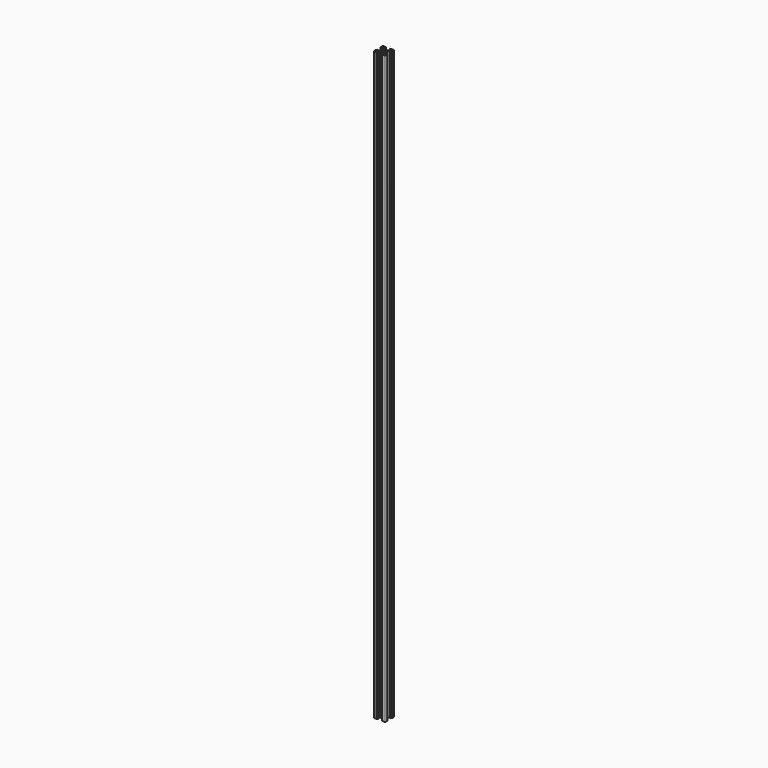
from build123d import *

# Parameters (mm, degrees)
F0_R     = 2.09999979
F1_DEPTH = 1000


# Not quite as in the source:
# - ends of sketch curves that miss each other by under 0.0002 mm in the source are joined


with BuildPart() as f1:
    # F0 (on Top) → F1 (new body)
    with BuildSketch(Plane.XY):
        with BuildLine():
            Line((-4.639999536, 10), (-8.50000015, 10))
            ThreePointArc((-8.50000015, 10), (-9.5606602157, 9.5606602157), (-10, 8.50000015))
            Line((-10, 8.50000015), (-10, 4.639999536))
            Line((-10, 4.639999536), (-8.19999818, 2.839999716))
            Line((-8.19999818, 2.839999716), (-8.19999818, 5.4993384501))
            Line((-8.19999818, 5.4993384501), (-6.559999344, 5.4993384501))
            Line((-6.559999344, 5.4993384501), (-3.9006596099, 2.839999716))
            Line((-3.9006596099, 2.839999716), (-3.9006596099, 0.19999898))
            Line((-3.9006596099, 0.19999898), (-3.7006596299, -1e-06))
            Line((-3.7006596299, -1e-06), (-3.9006596099, -0.20000098))
            Line((-3.9006596099, -0.20000098), (-3.9006596099, -2.840000716))
            Line((-3.9006596099, -2.840000716), (-6.559999344, -5.4993404501))
            Line((-6.559999344, -5.4993404501), (-8.19999818, -5.4993404501))
            Line((-8.19999818, -5.4993404501), (-8.19999818, -2.840000716))
            Line((-8.19999818, -2.840000716), (-10, -4.640000536))
            Line((-10, -4.640000536), (-10, -8.50000115))
            ThreePointArc((-10, -8.50000115), (-9.5606602157, -9.5606612157), (-8.50000015, -10.000001))
            Line((-8.50000015, -10.000001), (-4.639999536, -10))
            Line((-4.639999536, -10), (-2.839999716, -8.20000018))
            Line((-2.839999716, -8.20000018), (-5.4993394501, -8.20000018))
            Line((-5.4993394501, -8.20000018), (-5.4993394501, -6.560000344))
            Line((-5.4993394501, -6.560000344), (-2.839999716, -3.9006606099))
            Line((-2.839999716, -3.9006606099), (-0.19999898, -3.9006606099))
            Line((-0.19999898, -3.9006606099), (1e-06, -3.7006606299))
            Line((1e-06, -3.7006606299), (0.20000098, -3.9006606099))
            Line((0.20000098, -3.9006606099), (2.839999716, -3.9006606099))
            Line((2.839999716, -3.9006606099), (5.4993414501, -6.560000344))
            Line((5.4993414501, -6.560000344), (5.4993414501, -8.20000018))
            Line((5.4993414501, -8.20000018), (2.839999716, -8.20000018))
            Line((2.839999716, -8.20000018), (4.639999536, -10))
            Line((4.639999536, -10), (8.50000015, -10))
            ThreePointArc((8.50000015, -10), (9.5606602157, -9.5606612157), (10, -8.50000115))
            Line((10, -8.50000115), (10, -4.640000536))
            Line((10, -4.640000536), (8.20000018, -2.840000716))
            Line((8.20000018, -2.840000716), (8.20000018, -5.4993404501))
            Line((8.20000018, -5.4993404501), (6.560000344, -5.4993404501))
            Line((6.560000344, -5.4993404501), (3.9006596099, -2.840000716))
            Line((3.9006596099, -2.840000716), (3.9006596099, -0.20000098))
            Line((3.9006596099, -0.20000098), (3.7006596299, -1e-06))
            Line((3.7006596299, -1e-06), (3.9006596099, 0.19999898))
            Line((3.9006596099, 0.19999898), (3.9006596099, 2.839999716))
            Line((3.9006596099, 2.839999716), (6.560000344, 5.4993384501))
            Line((6.560000344, 5.4993384501), (8.20000018, 5.4993384501))
            Line((8.20000018, 5.4993384501), (8.20000018, 2.839999716))
            Line((8.20000018, 2.839999716), (10, 4.639999536))
            Line((10, 4.639999536), (10, 8.50000015))
            ThreePointArc((10, 8.50000015), (9.5606602157, 9.5606602157), (8.50000015, 10))
            Line((8.50000015, 10), (4.639999536, 10))
            Line((4.639999536, 10), (2.839999716, 8.20000018))
            Line((2.839999716, 8.20000018), (5.4993414501, 8.20000018))
            Line((5.4993414501, 8.20000018), (5.4993414501, 6.559998344))
            Line((5.4993414501, 6.559998344), (2.839999716, 3.9006596099))
            Line((2.839999716, 3.9006596099), (0.20000098, 3.9006596099))
            Line((0.20000098, 3.9006596099), (1e-06, 3.7006596299))
            Line((1e-06, 3.7006596299), (-0.19999898, 3.9006596099))
            Line((-0.19999898, 3.9006596099), (-2.839999716, 3.9006596099))
            Line((-2.839999716, 3.9006596099), (-5.4993394501, 6.559998344))
            Line((-5.4993394501, 6.559998344), (-5.4993394501, 8.20000018))
            Line((-5.4993394501, 8.20000018), (-2.839999716, 8.20000018))
            Line((-2.839999716, 8.20000018), (-4.639999536, 10))
        make_face()
        Polygon((-6.5693393431, -8.20000018), (-8.19999818, -8.20000018), (-8.19999818, -6.5693403431), (-7.629998237, -6.5693403431), (-6.5693393431, -7.630000237), align=None, mode=Mode.SUBTRACT)
        Polygon((8.20000018, -8.20000018), (6.5693393431, -8.20000018), (6.5693393431, -7.630000237), (7.630002237, -6.5693403431), (8.20000018, -6.5693403431), align=None, mode=Mode.SUBTRACT)
        with Locations((1e-06, -1e-06)):
            Circle(F0_R, mode=Mode.SUBTRACT)
        Polygon((-8.19999818, 8.20000018), (-6.5693393431, 8.20000018), (-6.5693393431, 7.629999237), (-7.629998237, 6.5693393431), (-8.19999818, 6.5693393431), align=None, mode=Mode.SUBTRACT)
        Polygon((6.5693393431, 8.20000018), (8.20000018, 8.20000018), (8.20000018, 6.5693393431), (7.630002237, 6.5693393431), (6.5693393431, 7.629999237), align=None, mode=Mode.SUBTRACT)
    extrude(amount=F1_DEPTH)


solid = f1.part
